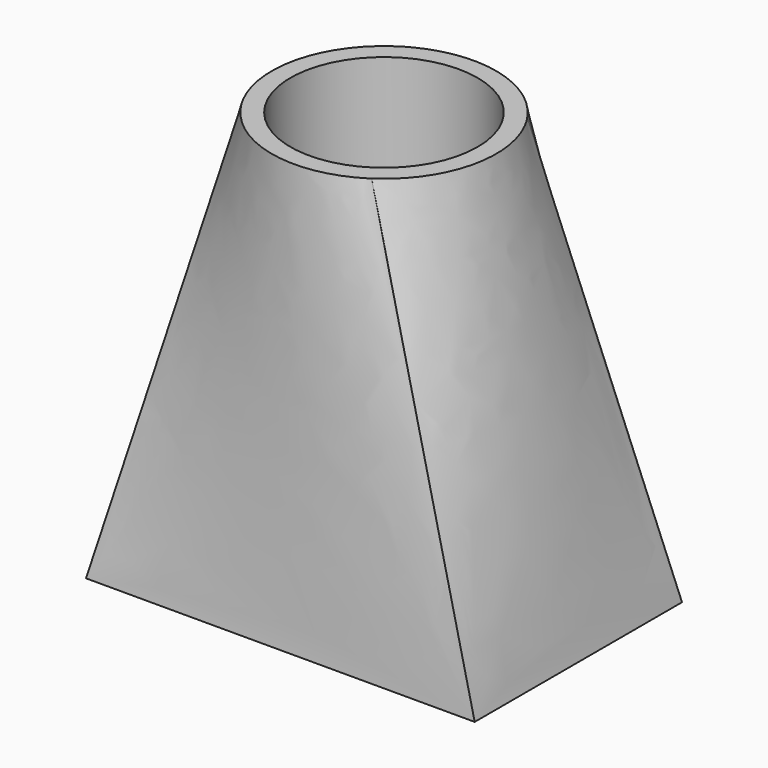
from build123d import *

# Parameters (mm, degrees)
F5_W     = 93.8750132918
F5_H     = 62.5833421946
F7_R     = 22.6051057699
F8_DEPTH = 93.98


# Not quite as in the source:
# - the arcs of a loft's sections are written as splines that run evenly, so that the points pair up as in the source's solid
# - the program builds the solid bodies; features that only make, move or delete a surface that nothing else refers to are left out


with BuildPart() as f6:
    # F5 (on Top) → F6 section 0
    with BuildSketch(Plane.XY):
        Rectangle(F5_W, F5_H)
    # F4 (on offset) → F6 section 1
    with BuildSketch(Plane.XY.offset(101.6)):
        with BuildLine():
            add(Edge.make_bspline(
                [(22.5525184305, 15.035012287), (21.5684791775, 16.5110711666), (20.439088741, 17.8901765373), (17.9328967072, 20.4016171121), (16.5561570804, 21.5338902158), (13.6081630734, 23.5081403532), (12.0369815881, 24.3500685697), (8.7604753642, 25.7112589441), (7.0552316437, 26.2304874441), (3.5761274997, 26.9263082729), (1.8023531039, 27.1028833962), (-1.7456489391, 27.1065946751), (-3.519788855, 26.9337307389), (-7.0003410682, 26.2451898455), (-8.706667302, 25.7295299139), (-11.9860140158, 24.3751970887), (-13.5589534074, 23.5365576836), (-15.035012287, 22.5525184305)],
                knots=[0, 0, 0, 0, 0.125, 0.125, 0.25, 0.25, 0.375, 0.375, 0.5, 0.5, 0.625, 0.625, 0.75, 0.75, 0.875, 0.875, 1, 1, 1, 1], degree=3))
            add(Edge.make_bspline(
                [(-15.035012287, 22.5525184305), (-16.5110711666, 21.5684791775), (-17.8901765373, 20.439088741), (-20.4016171121, 17.9328967072), (-21.5338902158, 16.5561570804), (-23.5081403532, 13.6081630734), (-24.3500685697, 12.0369815881), (-25.7112589441, 8.7604753642), (-26.2304874441, 7.0552316437), (-26.9263082729, 3.5761274997), (-27.1028833962, 1.8023531039), (-27.1065946751, -1.7456489391), (-26.9337307389, -3.519788855), (-26.2451898455, -7.0003410682), (-25.7295299139, -8.706667302), (-24.3751970887, -11.9860140158), (-23.5365576836, -13.5589534074), (-22.5525184305, -15.035012287)],
                knots=[0, 0, 0, 0, 0.125, 0.125, 0.25, 0.25, 0.375, 0.375, 0.5, 0.5, 0.625, 0.625, 0.75, 0.75, 0.875, 0.875, 1, 1, 1, 1], degree=3))
            add(Edge.make_bspline(
                [(-22.5525184305, -15.035012287), (-21.5684791775, -16.5110711666), (-20.439088741, -17.8901765373), (-17.9328967072, -20.4016171121), (-16.5561570804, -21.5338902158), (-13.6081630734, -23.5081403532), (-12.0369815881, -24.3500685697), (-8.7604753642, -25.7112589441), (-7.0552316437, -26.2304874441), (-3.5761274997, -26.9263082729), (-1.8023531039, -27.1028833962), (1.7456489391, -27.1065946751), (3.519788855, -26.9337307389), (7.0003410682, -26.2451898455), (8.706667302, -25.7295299139), (11.9860140158, -24.3751970887), (13.5589534074, -23.5365576836), (15.035012287, -22.5525184305)],
                knots=[0, 0, 0, 0, 0.125, 0.125, 0.25, 0.25, 0.375, 0.375, 0.5, 0.5, 0.625, 0.625, 0.75, 0.75, 0.875, 0.875, 1, 1, 1, 1], degree=3))
            add(Edge.make_bspline(
                [(15.035012287, -22.5525184305), (16.5110711666, -21.5684791775), (17.8901765373, -20.439088741), (20.4016171121, -17.9328967072), (21.5338902158, -16.5561570804), (23.5081403532, -13.6081630734), (24.3500685697, -12.0369815881), (25.7112589441, -8.7604753642), (26.2304874441, -7.0552316437), (26.9263082729, -3.5761274997), (27.1028833962, -1.8023531039), (27.1065946751, 1.7456489391), (26.9337307389, 3.519788855), (26.2451898455, 7.0003410682), (25.7295299139, 8.706667302), (24.3751970887, 11.9860140158), (23.5365576836, 13.5589534074), (22.5525184305, 15.035012287)],
                knots=[0, 0, 0, 0, 0.125, 0.125, 0.25, 0.25, 0.375, 0.375, 0.5, 0.5, 0.625, 0.625, 0.75, 0.75, 0.875, 0.875, 1, 1, 1, 1], degree=3))
        make_face()
    loft(ruled=True)

    # F7 (on offset) → F8 (cut)
    with BuildSketch(Plane.XY.offset(101.6)):
        Circle(F7_R)
    extrude(amount=-F8_DEPTH, mode=Mode.SUBTRACT)


solid = f6.part
